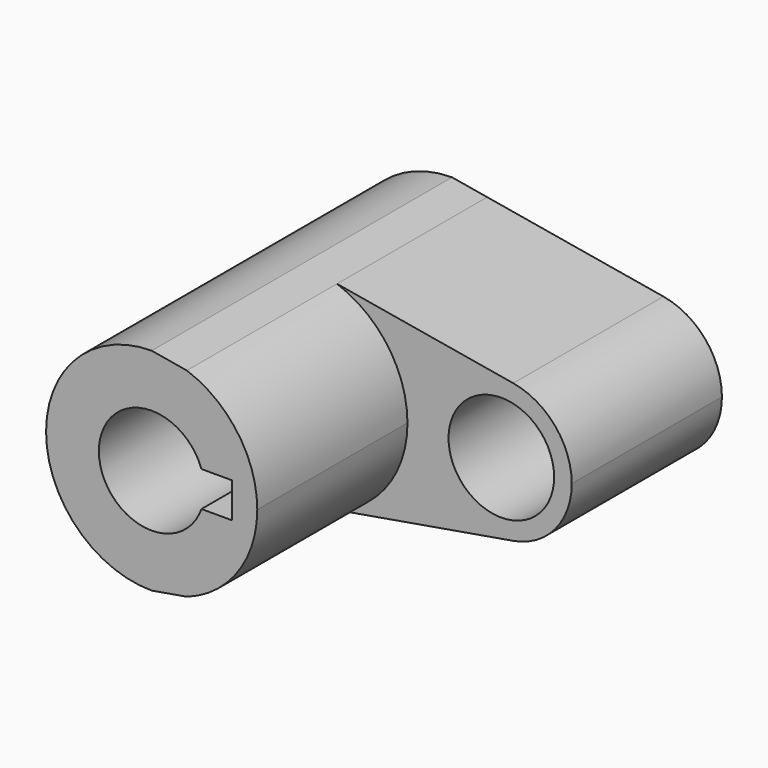
from build123d import *

# Parameters (mm, degrees)
F0_R     = 14.2875
F1_DEPTH = 50.8
F2_DEPTH = 101.6


with BuildPart() as f1:
    # F0 (on Front) → F1 (new body)
    with BuildSketch(Plane.XZ):
        with BuildLine():
            Line((9.5121844836, 26.9452959039), (0, 28.575))
            ThreePointArc((0, 28.575), (-28.575, 0), (0, -28.575))
            Line((0, -28.575), (9.5121844836, -26.9452959039))
            ThreePointArc((9.5121844836, -26.9452959039), (23.3274655355, -16.5033322905), (28.575, 0))
            ThreePointArc((28.575, 0), (23.3274655355, 16.5033322905), (9.5121844836, 26.9452959039))
        make_face()
        with BuildLine():
            ThreePointArc((-13.4703841816, 4.7625), (0, 14.2875), (13.4703841816, 4.7625))
            Line((13.4703841816, 4.7625), (21.7597242445, 4.7625))
            Line((21.7597242445, 4.7625), (21.7597242445, -4.7625))
            Line((21.7597242445, -4.7625), (13.4703841816, -4.7625))
            ThreePointArc((13.4703841816, -4.7625), (0, -14.2875), (-13.4703841816, -4.7625))
            Line((-13.4703841816, -4.7625), (-21.7597242445, -4.7625))
            Line((-21.7597242445, -4.7625), (-21.7597242445, 4.7625))
            Line((-21.7597242445, 4.7625), (-13.4703841816, 4.7625))
        make_face(mode=Mode.SUBTRACT)
        with BuildLine():
            Line((57.1919272622, 18.7764181619), (9.5121844836, 26.9452959039))
            ThreePointArc((9.5121844836, 26.9452959039), (23.3274655355, 16.5033322905), (28.575, 0))
            ThreePointArc((28.575, 0), (23.3274655355, -16.5033322905), (9.5121844836, -26.9452959039))
            Line((9.5121844836, -26.9452959039), (57.1919272622, -18.7764181619))
            ThreePointArc((57.1919272622, -18.7764181619), (34.925, 0), (57.1919272622, 18.7764181619))
        make_face()
        with BuildLine():
            ThreePointArc((73.025, 0), (68.5383952831, 12.2804730295), (57.1919272622, 18.7764181619))
            ThreePointArc((57.1919272622, 18.7764181619), (34.925, 0), (57.1919272622, -18.7764181619))
            ThreePointArc((57.1919272622, -18.7764181619), (68.5383952831, -12.2804730295), (73.025, 0))
        make_face()
        with Locations((53.975, 0)):
            Circle(F0_R, mode=Mode.SUBTRACT)
        with BuildLine():
            ThreePointArc((-13.4703841816, -4.7625), (-14.2875, 0), (-13.4703841816, 4.7625))
            Line((-13.4703841816, 4.7625), (-21.7597242445, 4.7625))
            Line((-21.7597242445, 4.7625), (-21.7597242445, -4.7625))
            Line((-21.7597242445, -4.7625), (-13.4703841816, -4.7625))
        make_face()
    extrude(amount=F1_DEPTH)

    # F0 (on Front) → F2 (join)
    with BuildSketch(Plane.XZ):
        with BuildLine():
            Line((9.5121844836, 26.9452959039), (0, 28.575))
            ThreePointArc((0, 28.575), (-28.575, 0), (0, -28.575))
            Line((0, -28.575), (9.5121844836, -26.9452959039))
            ThreePointArc((9.5121844836, -26.9452959039), (23.3274655355, -16.5033322905), (28.575, 0))
            ThreePointArc((28.575, 0), (23.3274655355, 16.5033322905), (9.5121844836, 26.9452959039))
        make_face()
        with BuildLine():
            ThreePointArc((-13.4703841816, 4.7625), (0, 14.2875), (13.4703841816, 4.7625))
            Line((13.4703841816, 4.7625), (21.7597242445, 4.7625))
            Line((21.7597242445, 4.7625), (21.7597242445, -4.7625))
            Line((21.7597242445, -4.7625), (13.4703841816, -4.7625))
            ThreePointArc((13.4703841816, -4.7625), (0, -14.2875), (-13.4703841816, -4.7625))
            Line((-13.4703841816, -4.7625), (-21.7597242445, -4.7625))
            Line((-21.7597242445, -4.7625), (-21.7597242445, 4.7625))
            Line((-21.7597242445, 4.7625), (-13.4703841816, 4.7625))
        make_face(mode=Mode.SUBTRACT)
        with BuildLine():
            ThreePointArc((-13.4703841816, -4.7625), (-14.2875, 0), (-13.4703841816, 4.7625))
            Line((-13.4703841816, 4.7625), (-21.7597242445, 4.7625))
            Line((-21.7597242445, 4.7625), (-21.7597242445, -4.7625))
            Line((-21.7597242445, -4.7625), (-13.4703841816, -4.7625))
        make_face()
    extrude(amount=F2_DEPTH)


solid = f1.part
